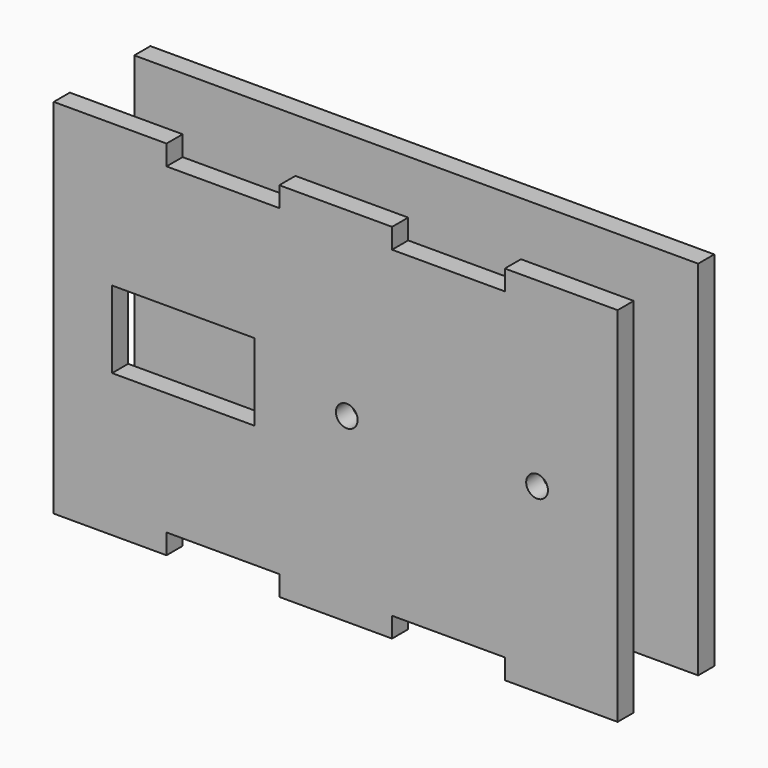
from build123d import *

# Parameters (mm, degrees)
F0_W       = 88.9
F0_H       = 3.175
F1_DEPTH   = 57.15
F2_W       = 17.78
F2_H       = 3.175
F2_W_2     = 22.479
F2_H_2     = 6.080125
F1_FACE1_W = 88.9
F1_FACE1_H = 57.15
F3_DEPTH   = 19.051


with BuildPart() as f1:
    # F0 (on Top) → F1 (new body)
    with BuildSketch(Plane.XY):
        with Locations((0, 7.9375)):
            Rectangle(F0_W, F0_H)
    extrude(amount=F1_DEPTH)


with BuildPart() as f1b:
    # F0 (on Top) → F1, piece 2 (new body)
    with BuildSketch(Plane.XY):
        with Locations((0, -7.9375)):
            Rectangle(F0_W, F0_H)
    extrude(amount=F1_DEPTH)

    # F2 (on face) + F1_face1 (on face) → F3 (cut, through all)
    with BuildSketch(Plane.XZ.offset(9.525)):
        with Locations((-17.78, 55.5625)):
            Rectangle(F2_W, F2_H)
        with Locations((17.78, 55.5625)):
            Rectangle(F2_W, F2_H)
        with Locations((-17.78, 1.5875)):
            Rectangle(F2_W, F2_H)
        with Locations((17.78, 1.5875)):
            Rectangle(F2_W, F2_H)
        with Locations((-24.0125088, 31.6150625)):
            Rectangle(F2_W_2, F2_H_2)
        with Locations((-24.0125088, 25.5349375)):
            Rectangle(F2_W_2, F2_H_2)
        with BuildLine():
            Line((3.4645, 28.575), (0.0355, 28.575))
            ThreePointArc((0.0355, 28.575), (1.75, 26.8605), (3.4645, 28.575))
        make_face()
        with BuildLine():
            ThreePointArc((3.4645, 28.575), (1.75, 30.2895), (0.0355, 28.575))
            Line((0.0355, 28.575), (3.4645, 28.575))
        make_face()
        with BuildLine():
            Line((33.4645, 28.575), (30.0355, 28.575))
            ThreePointArc((30.0355, 28.575), (31.75, 26.8605), (33.4645, 28.575))
        make_face()
        with BuildLine():
            ThreePointArc((33.4645, 28.575), (31.75, 30.2895), (30.0355, 28.575))
            Line((30.0355, 28.575), (33.4645, 28.575))
        make_face()
    with BuildSketch(Plane(origin=(0, -6.35, 28.575), x_dir=(-1, 0, 0), z_dir=(0, 1, 0))):
        Rectangle(F1_FACE1_W, F1_FACE1_H)
    extrude(amount=-F3_DEPTH, dir=(0, -1, 0), mode=Mode.SUBTRACT)


solid = Compound([f1.part, f1b.part])
